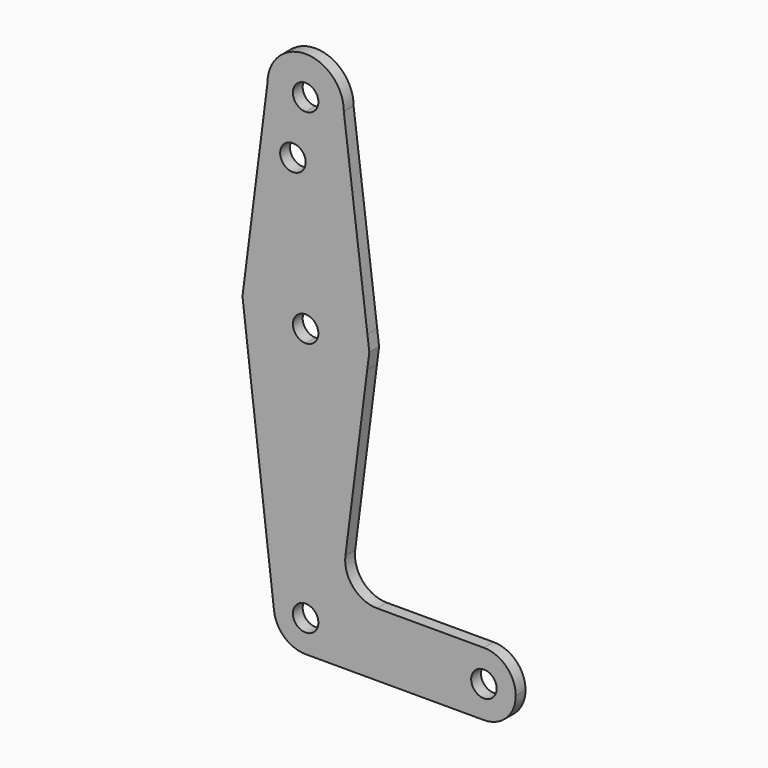
from build123d import *

# Parameters (mm, degrees)
F0_R     = 3.175
F1_DEPTH = 3.048


# Not quite as in the source:
# - a feature names something its author has since deleted; it is built from what else it names


with BuildPart() as f1:
    # F0 (on Front) → F1 (new body)
    with BuildSketch(Plane.XZ):
        with BuildLine():
            ThreePointArc((-9.524828548, 63.1542134468), (-6.7149560856, 56.455996051), (0, 53.6863635294))
            ThreePointArc((0, 53.6863635294), (6.7149544249, 56.4559944002), (9.5248285199, 63.1542087637))
            ThreePointArc((9.5248285199, 63.1542087637), (9.5249571299, 63.1827860179), (9.525, 63.2113635294))
            ThreePointArc((9.525, 63.2113635294), (-0.0285751699, 72.7363206663), (-9.524828548, 63.1542134468))
        make_face()
        with BuildLine():
            ThreePointArc((3.175, 63.2113635294), (2.2450640303, 60.9662994992), (0, 60.0363635294))
            ThreePointArc((0, 60.0363635294), (-2.2450640303, 65.4564275597), (3.175, 63.2113635294))
        make_face(mode=Mode.SUBTRACT)
        with BuildLine():
            ThreePointArc((9.5248285199, 63.1542087637), (6.7149544249, 56.4559944002), (0, 53.6863635294))
            Line((0, 53.6863635294), (0, 48.9365635294))
            Line((0, 48.9365635294), (0, 28.2863635294))
            ThreePointArc((0, 28.2863635294), (9.7569068314, 24.9340786537), (15.3931294165, 16.2930116029))
            Line((15.3931294165, 16.2930116029), (9.5248285199, 63.1542087637))
        make_face()
        with BuildLine():
            Line((0, 48.9365635294), (0, 53.6863635294))
            ThreePointArc((0, 53.6863635294), (-6.7149560856, 56.455996051), (-9.524828548, 63.1542134468))
            Line((-9.524828548, 63.1542134468), (-15.7471542329, 14.4220247552))
            ThreePointArc((-15.7471542329, 14.4220247552), (-10.4903855516, 24.3263723829), (0, 28.2863635294))
            Line((0, 28.2863635294), (0, 48.9365635294))
        make_face()
        with Locations((-3.175, 48.9365635294)):
            Circle(F0_R, mode=Mode.SUBTRACT)
        with BuildLine():
            ThreePointArc((15.3931294165, 16.2930116029), (9.7569068314, 24.9340786537), (0, 28.2863635294))
            Line((0, 28.2863635294), (0, 15.5863635294))
            ThreePointArc((0, 15.5863635294), (2.2450640303, 14.6564275597), (3.175, 12.4113635294))
            ThreePointArc((3.175, 12.4113635294), (2.2450640303, 10.1662994992), (0, 9.2363635294))
            Line((0, 9.2363635294), (0, -3.4636364706))
            ThreePointArc((0, -3.4636364706), (9.6997269009, -0.1556935265), (15.3571050572, 8.3895543266))
            Line((15.3571050572, 8.3895543266), (15.8749636535, 12.445334128))
            Line((15.8749636535, 12.445334128), (15.3931294165, 16.2930116029))
        make_face()
        with BuildLine():
            Line((0, 15.5863635294), (0, 28.2863635294))
            ThreePointArc((0, 28.2863635294), (-10.4903855516, 24.3263723829), (-15.7471542329, 14.4220247552))
            Line((-15.7471542329, 14.4220247552), (-14.8425870633, 6.7799130706))
            ThreePointArc((-14.8425870633, 6.7799130706), (-9.017104551, -0.6541426038), (0, -3.4636364706))
            Line((0, -3.4636364706), (0, 9.2363635294))
            ThreePointArc((0, 9.2363635294), (-3.175, 12.4113635294), (0, 15.5863635294))
        make_face()
        with BuildLine():
            ThreePointArc((0, -3.4636364706), (-9.017104551, -0.6541426038), (-14.8425870633, 6.7799130706))
            Line((-14.8425870633, 6.7799130706), (-7.8824732142, -52.0216543038))
            ThreePointArc((-7.8824732142, -52.0216543038), (-5.9333689967, -45.8161571108), (0, -43.1511364706))
            Line((0, -43.1511364706), (0, -3.4636364706))
        make_face()
        with BuildLine():
            ThreePointArc((15.3571050572, 8.3895543266), (9.6997269009, -0.1556935265), (0, -3.4636364706))
            Line((0, -3.4636364706), (0, -43.1511364706))
            ThreePointArc((0, -43.1511364706), (5.6126600757, -45.4759763949), (7.9375, -51.0886364706))
            Line((7.9375, -51.0886364706), (36.5125, -51.0886364706))
            ThreePointArc((36.5125, -51.0886364706), (38.8373399243, -45.4759763949), (44.45, -43.1511364706))
            Line((44.45, -43.1511364706), (17.8060374021, -43.1511364706))
            ThreePointArc((17.8060374021, -43.1511364706), (11.8390009683, -40.4545215548), (9.9198625623, -34.1939973287))
            Line((9.9198625623, -34.1939973287), (15.3571050572, 8.3895543266))
        make_face()
        with BuildLine():
            ThreePointArc((0, -43.1511364706), (-5.9333689967, -45.8161571108), (-7.8824732142, -52.0216543038))
            ThreePointArc((-7.8824732142, -52.0216543038), (-5.2724793598, -57.0220054673), (0, -59.0261364706))
            ThreePointArc((0, -59.0261364706), (5.6126600757, -56.7012965462), (7.9375, -51.0886364706))
            Line((7.9375, -51.0886364706), (3.175, -51.0886364706))
            ThreePointArc((3.175, -51.0886364706), (-2.2450640303, -53.3337005008), (0, -47.9136364706))
            Line((0, -47.9136364706), (0, -43.1511364706))
        make_face()
        with BuildLine():
            ThreePointArc((7.9375, -51.0886364706), (5.6126600757, -45.4759763949), (0, -43.1511364706))
            Line((0, -43.1511364706), (0, -47.9136364706))
            ThreePointArc((0, -47.9136364706), (2.2450640303, -48.8435724403), (3.175, -51.0886364706))
            Line((3.175, -51.0886364706), (7.9375, -51.0886364706))
        make_face()
        with BuildLine():
            ThreePointArc((7.9375, -51.0886364706), (5.6126600757, -56.7012965462), (0, -59.0261364706))
            Line((0, -59.0261364706), (44.45, -59.0261364706))
            ThreePointArc((44.45, -59.0261364706), (38.8373399243, -56.7012965462), (36.5125, -51.0886364706))
            Line((36.5125, -51.0886364706), (7.9375, -51.0886364706))
        make_face()
        with BuildLine():
            ThreePointArc((36.5125, -51.0886364706), (38.8373399243, -56.7012965462), (44.45, -59.0261364706))
            ThreePointArc((44.45, -59.0261364706), (50.0626600757, -56.7012965462), (52.3875, -51.0886364706))
            ThreePointArc((52.3875, -51.0886364706), (50.0626600757, -45.4759763949), (44.45, -43.1511364706))
            ThreePointArc((44.45, -43.1511364706), (38.8373399243, -45.4759763949), (36.5125, -51.0886364706))
        make_face()
        with BuildLine():
            ThreePointArc((47.625, -51.0886364706), (44.45, -54.2636364706), (41.275, -51.0886364706))
            ThreePointArc((41.275, -51.0886364706), (44.45, -47.9136364706), (47.625, -51.0886364706))
        make_face(mode=Mode.SUBTRACT)
    extrude(amount=F1_DEPTH)


solid = f1.part
